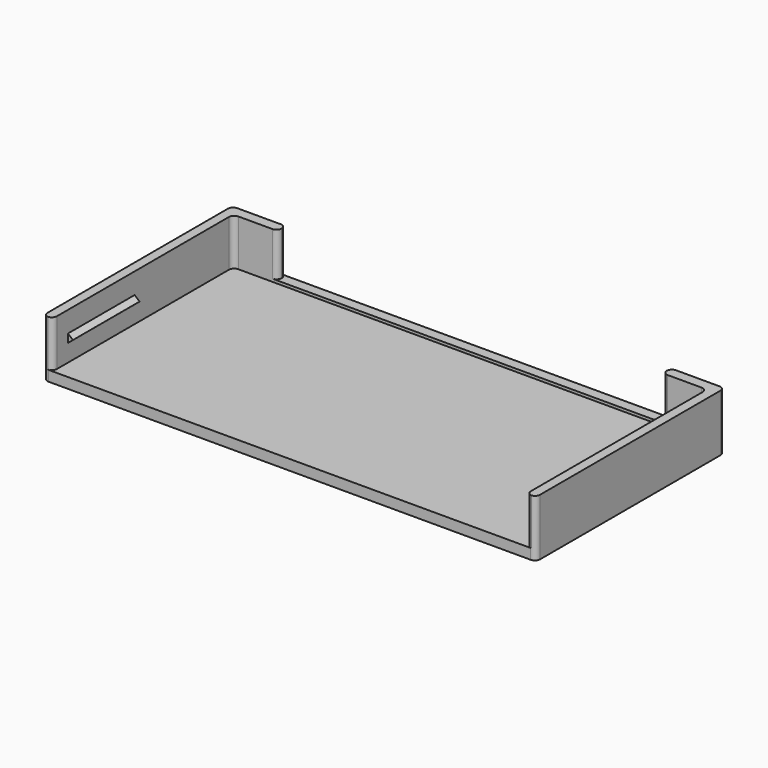
from build123d import *

# Parameters (mm, degrees)
F1_DEPTH     = 3
F0_W         = 2.7
F0_H         = 65
F2_DEPTH     = 16.4
F0_W_2       = 111
F0_H_2       = 3
F3_DEPTH     = 3.8
F4_W         = 24
F4_H         = 2.4
F5_DEPTH     = 1.5
F6_W         = 24
F6_H         = 2.4
F7_DEPTH     = 1.5
F8_T1_DEPTH  = 31.73221831
F8_T6_DEPTH  = 31.73221831
F8_T11_DEPTH = 31.73221831
F8_T16_DEPTH = 31.73221831
F9_F1_R      = 1.5
F9_F2_R      = 1.5
F9_F3_R      = 1.4999
F9_F4_R      = 1.4999
F9_F5_R      = 1.5
F9_F6_R      = 1.5
F9_F7_R      = 1.5
F9_F8_R      = 1.5
F9_F9_R      = 1.5
F9_F10_R     = 1.5
F9_F11_R     = 1.5
F9_F12_R     = 1.5


# Not quite as in the source:
# - a fillet or chamfer that OpenCascade refuses, or shapes differently, is made with other operations: its cross-section is extruded or revolved along the edge and cut away or added
# - a fillet or chamfer is up to 0.001 mm smaller than in the source, because OpenCascade refuses the exact size


with BuildPart() as f1:
    # F0 (on Top) → F1 (new body)
    with BuildSketch(Plane.XY):
        Polygon((-68.3, -32.5), (68.3, -32.5), (68.3, 32.5), (55.5, 32.5), (-55.5, 32.5), (-68.3, 32.5), align=None)
    extrude(amount=F1_DEPTH)

    # F0 (on Top) → F2 (join)
    with BuildSketch(Plane.XY):
        Polygon((-71, 32.5), (-68.3, 32.5), (-55.5, 32.5), (-55.5, 35.5), (-71, 35.5), align=None)
        with Locations((-69.65, 0)):
            Rectangle(F0_W, F0_H)
        Polygon((68.3, 32.5), (71, 32.5), (71, 35.5), (55.5, 35.5), (55.5, 32.5), align=None)
        with Locations((69.65, 0)):
            Rectangle(F0_W, F0_H)
    extrude(amount=F2_DEPTH)

    # F0 (on Top) → F3 (join)
    with BuildSketch(Plane.XY):
        with Locations((0, 34)):
            Rectangle(F0_W_2, F0_H_2)
    extrude(amount=F3_DEPTH)

    # F4 (on face) → F5 (join)
    with BuildSketch(Plane.YZ.offset(-68.3)):
        with Locations((-15, 9.2)):
            Rectangle(F4_W, F4_H)
    extrude(amount=F5_DEPTH)

    # F6 (on face) → F7 (join)
    with BuildSketch(Plane(origin=(68.3, 0, 0), x_dir=(0, -1, 0), z_dir=(-1, 0, 0))):
        with Locations((15, 9.2)):
            Rectangle(F6_W, F6_H)
    extrude(amount=F7_DEPTH)

    # F8: chamfer of 1.5 x 1.2586494468 on 4 edges, made by hand

    # F8_s2 → F8_t1 (cut)
    with BuildSketch(Plane.XZ.offset(-0.866109155)):
        Polygon((68.0586494468, 8), (66.8, 9.5), (66.8, 8), align=None)
    extrude(amount=F8_T1_DEPTH, mode=Mode.SUBTRACT)


with BuildPart() as f8_tool4:
    # F8_s5 → F8_t6 (new body)
    with BuildSketch(Plane.XZ.offset(-0.866109155)):
        Polygon((-68.3, 10.4), (-66.8, 9.1413505532), (-66.8, 10.4), align=None)
    extrude(amount=F8_T6_DEPTH)

    split(bisect_by=Plane.YZ.offset(-68.3), keep=Keep.TOP)


with BuildPart() as f1_1:
    add(f1.part)

    # F8_t3: cut F8_tool4
    add(f8_tool4.part, mode=Mode.SUBTRACT)


with BuildPart() as f8_tool9:
    # F8_s10 → F8_t11 (new body)
    with BuildSketch(Plane.XZ.offset(30.866109155)):
        Polygon((68.3, 10.4), (66.8, 9.1413505532), (66.8, 10.4), align=None)
    extrude(amount=-F8_T11_DEPTH)

    split(bisect_by=Plane.YZ.offset(68.3), keep=Keep.BOTTOM)


with BuildPart() as f1_2:
    add(f1_1.part)

    # F8_t8: cut F8_tool9
    add(f8_tool9.part, mode=Mode.SUBTRACT)


with BuildPart() as f8_tool14:
    # F8_s15 → F8_t16 (new body)
    with BuildSketch(Plane.XZ.offset(30.866109155)):
        Polygon((-68.3, 8), (-66.8, 9.2586494468), (-66.8, 8), align=None)
    extrude(amount=-F8_T16_DEPTH)

    split(bisect_by=Plane.YZ.offset(-68.3), keep=Keep.TOP)


with BuildPart() as f1_3:
    add(f1_2.part)

    # F8_t13: cut F8_tool14
    add(f8_tool14.part, mode=Mode.SUBTRACT)

    # F9: fillet of radius 1.5 on 12 edges, made by hand

    # F9_f1
    f9_f1_edges = [f1_3.edges().sort_by_distance(p)[0] for p in [
        (55.5, 35.5, 10.1),
    ]]
    fillet(f9_f1_edges, radius=F9_F1_R)

    # F9_f2
    f9_f2_edges = [f1_3.edges().sort_by_distance(p)[0] for p in [
        (-55.5, 35.5, 10.1),
    ]]
    fillet(f9_f2_edges, radius=F9_F2_R)

    # F9_f3 (radius 1.5 in the source; OpenCascade refuses exactly that, so slightly less here)
    f9_f3_edges = [f1_3.edges().sort_by_distance(p)[0] for p in [
        (-55.5, 32.5, 10.1),
    ]]
    fillet(f9_f3_edges, radius=F9_F3_R)

    # F9_f4 (radius 1.5 in the source; OpenCascade refuses exactly that, so slightly less here)
    f9_f4_edges = [f1_3.edges().sort_by_distance(p)[0] for p in [
        (55.5, 32.5, 10.1),
    ]]
    fillet(f9_f4_edges, radius=F9_F4_R)

    # F9_f5
    f9_f5_edges = [f1_3.edges().sort_by_distance(p)[0] for p in [
        (-68.3, -32.5, 9.7),
    ]]
    fillet(f9_f5_edges, radius=F9_F5_R)

    # F9_f6
    f9_f6_edges = [f1_3.edges().sort_by_distance(p)[0] for p in [
        (68.3, -32.5, 9.7),
    ]]
    fillet(f9_f6_edges, radius=F9_F6_R)

    # F9_f7
    f9_f7_edges = [f1_3.edges().sort_by_distance(p)[0] for p in [
        (-68.3, 32.5, 9.7),
    ]]
    fillet(f9_f7_edges, radius=F9_F7_R)

    # F9_f8
    f9_f8_edges = [f1_3.edges().sort_by_distance(p)[0] for p in [
        (68.3, 32.5, 9.7),
    ]]
    fillet(f9_f8_edges, radius=F9_F8_R)

    # F9_f9
    f9_f9_edges = [f1_3.edges().sort_by_distance(p)[0] for p in [
        (-71, -32.5, 8.2),
    ]]
    fillet(f9_f9_edges, radius=F9_F9_R)

    # F9_f10
    f9_f10_edges = [f1_3.edges().sort_by_distance(p)[0] for p in [
        (71, -32.5, 8.2),
    ]]
    fillet(f9_f10_edges, radius=F9_F10_R)

    # F9_f11
    f9_f11_edges = [f1_3.edges().sort_by_distance(p)[0] for p in [
        (-71, 35.5, 8.2),
    ]]
    fillet(f9_f11_edges, radius=F9_F11_R)

    # F9_f12
    f9_f12_edges = [f1_3.edges().sort_by_distance(p)[0] for p in [
        (71, 35.5, 8.2),
    ]]
    fillet(f9_f12_edges, radius=F9_F12_R)


solid = f1_3.part
